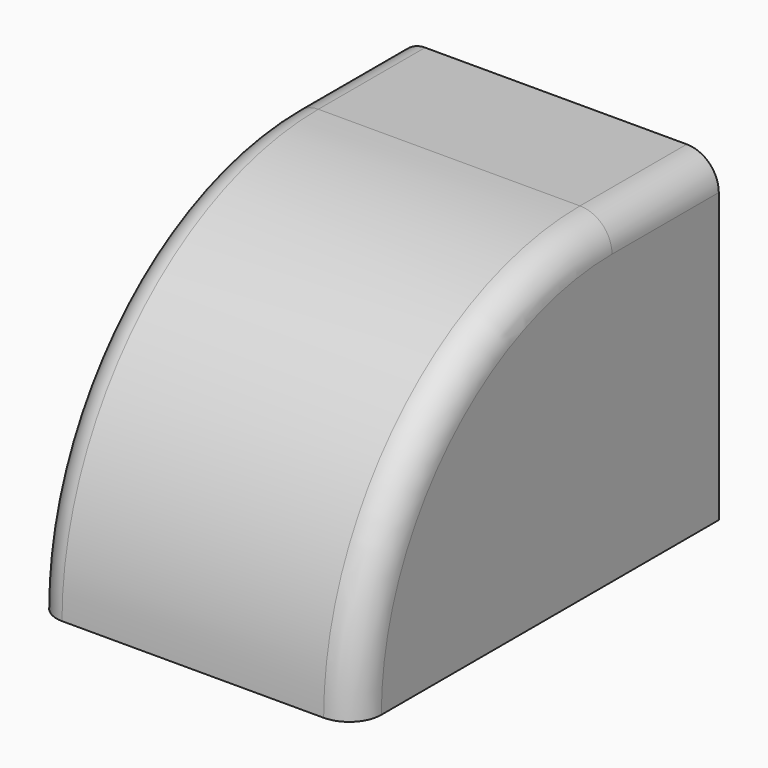
from build123d import *

# Parameters (mm, degrees)
F0_R        = 3
F0_R_2      = 17.0466335339
F1_DEPTH    = 25
F0_R_3      = 7.612861108
F1_FACE_R   = 3
F1_FACE_R_2 = 17.0466335339
F2_ANGLE    = 90
F1_FACE_R_3 = 7.612861108
F3_R        = 5


with BuildPart() as f1:
    # F0 (on Front) → F1 (new body)
    with BuildSketch(Plane.XZ):
        with BuildLine():
            Line((24, 30), (-30, 30))
            Line((-30, 30), (-30, -30))
            Line((-30, -30), (30, -30))
            Line((30, -30), (30, 24))
            ThreePointArc((30, 24), (28.2426406871, 28.2426406871), (24, 30))
        make_face()
        with Locations((-20, -20)):
            Circle(F0_R, mode=Mode.SUBTRACT)
        with Locations((20, -20)):
            Circle(F0_R, mode=Mode.SUBTRACT)
        with Locations((-20, 20)):
            Circle(F0_R, mode=Mode.SUBTRACT)
        Circle(F0_R_2, mode=Mode.SUBTRACT)
        with Locations((20, 20)):
            Circle(F0_R, mode=Mode.SUBTRACT)
    extrude(amount=F1_DEPTH)

    # F1_face (on face) → F2 (revolve)
    with BuildSketch(Plane(origin=(-0.0862793444, -25, -0.0862793444), x_dir=(1, 0, 0), z_dir=(0, -1, 0))):
        with BuildLine():
            Line((24.0862793444, 30.0862793444), (-29.9137206556, 30.0862793444))
            Line((-29.9137206556, 30.0862793444), (-29.9137206556, -29.9137206556))
            Line((-29.9137206556, -29.9137206556), (30.0862793444, -29.9137206556))
            Line((30.0862793444, -29.9137206556), (30.0862793444, 24.0862793444))
            ThreePointArc((30.0862793444, 24.0862793444), (28.3289200315, 28.3289200315), (24.0862793444, 30.0862793444))
        make_face()
        with Locations((-19.9137206556, -19.9137206556)):
            Circle(F1_FACE_R, mode=Mode.SUBTRACT)
        with Locations((20.0862793444, -19.9137206556)):
            Circle(F1_FACE_R, mode=Mode.SUBTRACT)
        with Locations((-19.9137206556, 20.0862793444)):
            Circle(F1_FACE_R, mode=Mode.SUBTRACT)
        with Locations((0.0862793444, 0.0862793444)):
            Circle(F1_FACE_R_2, mode=Mode.SUBTRACT)
        with Locations((20.0862793444, 20.0862793444)):
            Circle(F1_FACE_R, mode=Mode.SUBTRACT)
    revolve(axis=Axis((0, -25, -30), (1, 0, 0)), revolution_arc=F2_ANGLE)

    # F3
    f3_edges = [f1.edges().sort_by_distance(p)[0] for p in [
        (-30, -67.426407, 12.426407),
        (-30, -12.5, 30),
    ]]
    fillet(f3_edges, radius=F3_R)


with BuildPart() as f1b:
    # F0 (on Front) → F1, piece 2 (new body)
    with BuildSketch(Plane.XZ):
        Circle(F0_R_3)
    extrude(amount=F1_DEPTH)


with BuildPart() as f2:
    # F1_face (on face) → F2, piece 2 (revolve)
    with BuildSketch(Plane(origin=(-0.0862793444, -25, -0.0862793444), x_dir=(1, 0, 0), z_dir=(0, -1, 0))):
        with Locations((0.0862793444, 0.0862793444)):
            Circle(F1_FACE_R_3)
    revolve(axis=Axis((0, -25, -30), (1, 0, 0)), revolution_arc=F2_ANGLE)


solid = Compound([f1.part, f1b.part, f2.part])
